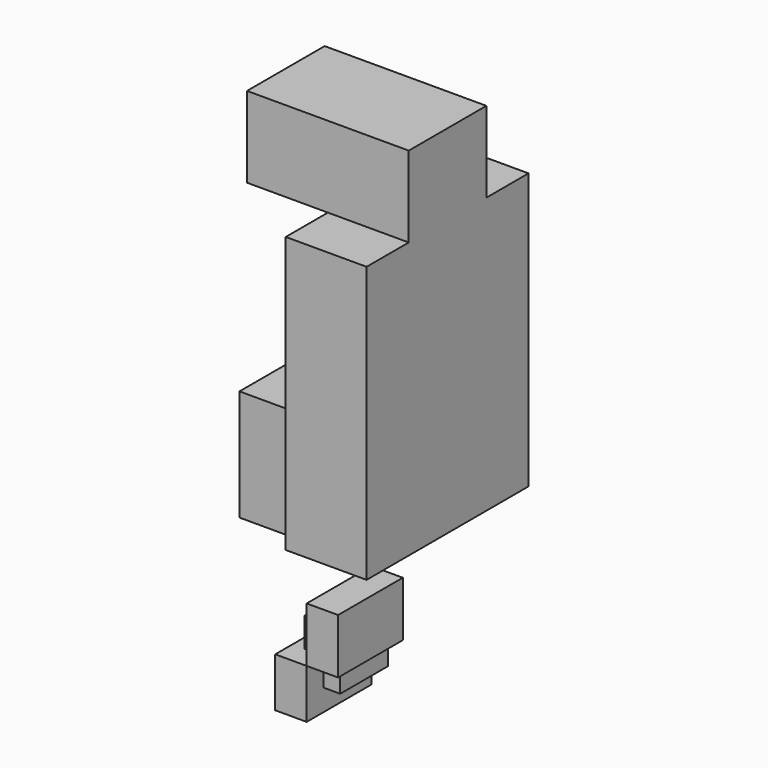
from build123d import *

# Parameters (mm, degrees)
F1_DEPTH  = 25
F0_W      = 5.9642354026
F0_H      = 9.0555474162
F2_DEPTH  = 18.4
F0_W_2    = 5.0806454383
F0_H_2    = 8.6162630469
F3_W      = 62.5787544996
F3_H      = 85.215434432
F4_DEPTH  = 25
F5_T      = -2.5
F6_W      = 57.5787544996
F6_H      = 34.3654131889
F7_DEPTH  = 38.8
F8_T      = -2.5
F9_W      = 25
F9_H      = 15
F10_DEPTH = 25
F11_W     = 30
F11_H     = 25
F12_DEPTH = 25


# Not quite as in the source:
# - a shell that OpenCascade refuses in one call is made with other operations: the cavity is built on its own and cut out


with BuildPart() as f1:
    # F0 (on Front) → F1 (new body)
    with BuildSketch(Plane.XZ):
        Polygon((0, 9.0555474162), (0, 0), (5.0806454383, 0), (9.7194965929, 0), (9.7194965929, 17.0078612864), (0, 17.0078612864), align=None)
    extrude(amount=F1_DEPTH)


with BuildPart() as f1b:
    # F0 (on Front) → F1, piece 2 (new body)
    with BuildSketch(Plane.XZ):
        Polygon((0, -8.6162630469), (0, 0), (-5.9642354026, 0), (-9.719, 0), (-9.719, -15.243191272), (0, -15.243191272), align=None)
    extrude(amount=F1_DEPTH)


with BuildPart() as f2:
    # F0 (on Front) → F2 (new body)
    with BuildSketch(Plane.XZ):
        with Locations((-2.9821177013, 4.5277737081)):
            Rectangle(F0_W, F0_H)
    extrude(amount=F2_DEPTH)


with BuildPart() as f2b:
    # F0 (on Front) → F2, piece 2 (new body)
    with BuildSketch(Plane.XZ):
        with Locations((2.5403227191, -4.3081315234)):
            Rectangle(F0_W_2, F0_H_2)
    extrude(amount=F2_DEPTH)


with BuildPart() as f4:
    # F3 (on Right) → F4 (new body)
    with BuildSketch(Plane.YZ):
        with Locations((-1.8009757623, 77.4449631572)):
            Rectangle(F3_W, F3_H)
    extrude(amount=F4_DEPTH)

    # F5
    f5_openings = [f4.faces().sort_by_distance(p)[0] for p in [
        (0, -1.800976, 77.444963),
    ]]
    offset(amount=F5_T, openings=f5_openings)

    # F6 (on face) → F7 (join)
    with BuildSketch(Plane(origin=(22.5, 0, 0), x_dir=(0, -1, 0), z_dir=(-1, 0, 0))):
        with Locations((1.8009757623, 54.5199525356)):
            Rectangle(F6_W, F6_H)
    extrude(amount=F7_DEPTH)

    # F8: a shell. OpenCascade refuses it in one call, so the cavity is built on its own and cut out:
    # the body offset inwards by the wall thickness, plus a prism from it out through each open face.
    f8_core = offset(f4.part, amount=F8_T, kind=Kind.INTERSECTION, mode=Mode.PRIVATE)
    f8_exits = [f8_core.faces().sort_by_distance(p)[0] for p in [
        (-13.8, -1.800976, 54.519953),
    ]]
    add(f8_core, mode=Mode.SUBTRACT)
    extrude(f8_exits, amount=-F8_T, mode=Mode.SUBTRACT)

    # F9 (on face) → F10 (join)
    with BuildSketch(Plane.XY.offset(120.0526803732)):
        with Locations((12.5, -9.3009757623)):
            Rectangle(F9_W, F9_H)
        with Locations((12.5, 5.6990242377)):
            Rectangle(F9_W, F9_H)
    extrude(amount=F10_DEPTH)

    # F11 (on face) → F12 (join)
    with BuildSketch(Plane(origin=(0, 0, 0), x_dir=(0, -1, 0), z_dir=(-1, 0, 0))):
        with Locations((1.8009757623, 132.5526803732)):
            Rectangle(F11_W, F11_H)
    extrude(amount=F12_DEPTH)


solid = Compound([f1.part, f1b.part, f2.part, f2b.part, f4.part])
